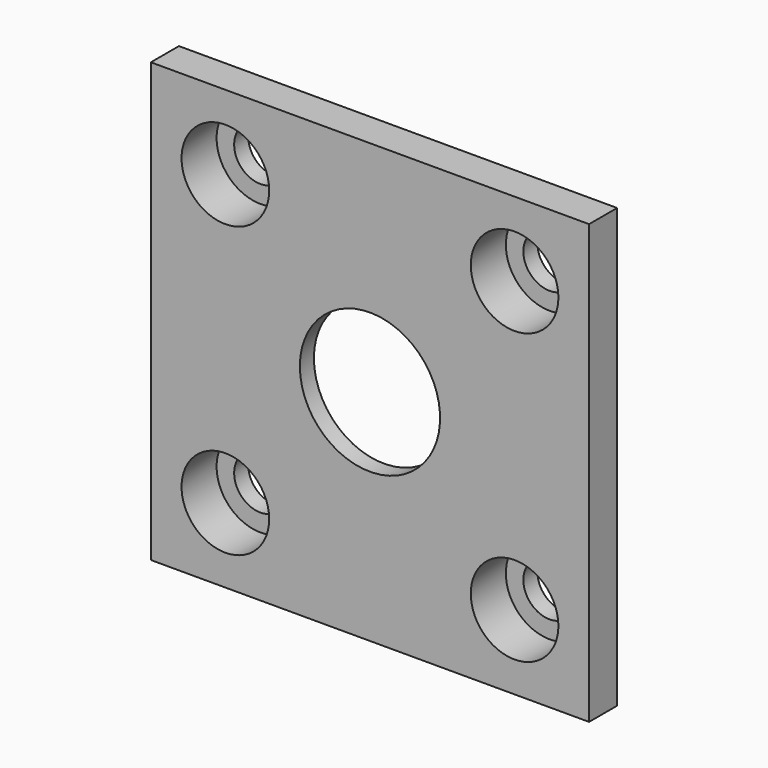
from build123d import *

# Parameters (mm, degrees)
F0_W      = 50
F0_H      = 50
F1_DEPTH  = 4
F2_W      = 44
F2_H      = 44
F3_DEPTH  = 3
F4_R      = 3
F5_DEPTH  = 25
F6_R      = 5
F6_R_2    = 3
F7_DEPTH  = 5
F8_R      = 16
F9_DEPTH  = 5
F10_R     = 8
F11_DEPTH = 25
F12_R     = 3


# Not quite as in the source:
# - a feature names something its author has since deleted; it is built from what else it names


with BuildPart() as f1:
    # F0 (on Front) → F1 (new body)
    with BuildSketch(Plane.XZ):
        Rectangle(F0_W, F0_H)
    extrude(amount=-F1_DEPTH)

    # F2 (on face) → F3 (join)
    with BuildSketch(Plane(origin=(0, 4, 0), x_dir=(-1, 0, 0), z_dir=(0, 1, 0))):
        Rectangle(F2_W, F2_H)
    extrude(amount=F3_DEPTH)

    # F4 (on face) → F5 (cut)
    with BuildSketch(Plane(origin=(0, 7, 0), x_dir=(-1, 0, 0), z_dir=(0, 1, 0))):
        with Locations((-16.5, 16.5)):
            Circle(F4_R)
        with Locations((16.5, 16.5)):
            Circle(F4_R)
        with Locations((16.5, -16.5)):
            Circle(F4_R)
        with Locations((-16.5, -16.5)):
            Circle(F4_R)
    extrude(amount=-F5_DEPTH, mode=Mode.SUBTRACT)

    # F6 (on face) → F7 (cut)
    with BuildSketch(Plane.XZ):
        with Locations((-16.5, 16.5)):
            Circle(F6_R)
        with Locations((-16.5, 16.5)):
            Circle(F6_R_2, mode=Mode.SUBTRACT)
        with Locations((16.5, 16.5)):
            Circle(F6_R)
        with Locations((16.5, 16.5)):
            Circle(F6_R_2, mode=Mode.SUBTRACT)
        with Locations((16.5, -16.5)):
            Circle(F6_R)
        with Locations((16.5, -16.5)):
            Circle(F6_R_2, mode=Mode.SUBTRACT)
        with Locations((-16.5, -16.5)):
            Circle(F6_R)
        with Locations((-16.5, -16.5)):
            Circle(F6_R_2, mode=Mode.SUBTRACT)
    extrude(amount=-F7_DEPTH, mode=Mode.SUBTRACT)

    # F8 (on face) → F9 (cut)
    with BuildSketch(Plane(origin=(0, 7, 0), x_dir=(-1, 0, 0), z_dir=(0, 1, 0))):
        Circle(F8_R)
    extrude(amount=-F9_DEPTH, mode=Mode.SUBTRACT)

    # F10 (on face) → F11 (cut)
    with BuildSketch(Plane(origin=(0, 2, 0), x_dir=(-1, 0, 0), z_dir=(0, 1, 0))):
        Circle(F10_R)
    extrude(amount=-F11_DEPTH, mode=Mode.SUBTRACT)

    # F12
    f12_edges = [f1.edges().sort_by_distance(p)[0] for p in [
        (-22, 5.5, 22),
        (-22, 5.5, -22),
        (22, 5.5, -22),
        (22, 5.5, 22),
    ]]
    fillet(f12_edges, radius=F12_R)


solid = f1.part
